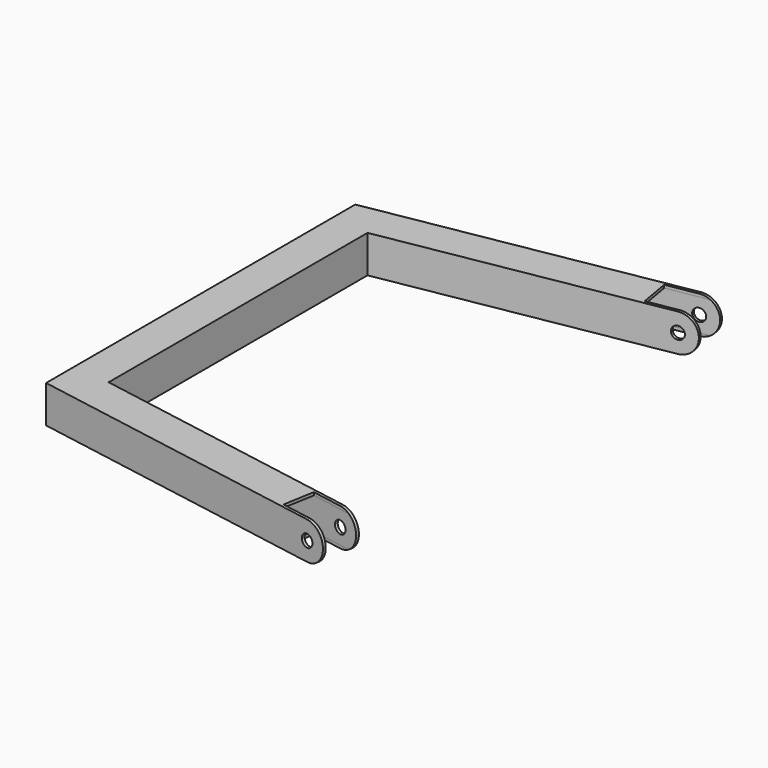
from build123d import *

# Parameters (mm, degrees)
F1_DEPTH  = 19.05
F2_T      = -1.4732
F3_W      = 16.1036
F3_H      = 19.05
F4_DEPTH  = 25.4
F5_R      = 9.52499
F6_R      = 3.175
F7_DEPTH  = 250.7881261572
F8_W      = 16.1036
F8_H      = 19.05
F9_DEPTH  = 25.4
F10_R     = 9.52499
F11_R     = 3.175
F12_DEPTH = 250.7881261572


# Not quite as in the source:
# - a fillet or chamfer is up to 0.001 mm smaller than in the source, because OpenCascade refuses the exact size


with BuildPart() as f1:
    # F0 (on Top) → F1 (new body)
    with BuildSketch(Plane.XY):
        Polygon((0, 225.425), (0, 28.575), (163.8898551464, 0), (167.1619531291, 18.766882394), (19.05, 44.5909277987), (19.05, 209.4090722013), (167.1619531291, 235.233117606), (163.8898551464, 254), align=None)
    extrude(amount=F1_DEPTH)

    # F2
    f2_openings = [f1.faces().sort_by_distance(p)[0] for p in [
        (165.525904, 9.383441, 9.525),
        (165.525904, 244.616559, 9.525),
    ]]
    offset(amount=F2_T, openings=f2_openings, kind=Kind.INTERSECTION)

    # F3 (on face) → F4 (cut)
    with BuildSketch(Plane(origin=(159.0546521525, -27.731958645, 0), x_dir=(0.1717636736, 0.9851381834, 0), z_dir=(0.9851381834, -0.1717636736, 0))):
        with Locations((37.6753235911, 9.525)):
            Rectangle(F3_W, F3_H)
    extrude(amount=-F4_DEPTH, mode=Mode.SUBTRACT)

    # F5 (radius 9.525 in the source; OpenCascade refuses exactly that, so slightly less here)
    f5_edges = [f1.edges().sort_by_distance(p)[0] for p in [
        (164.016376, 0.725653, 19.05),
        (167.035432, 18.04123, 19.05),
        (164.016376, 0.725653, 0),
        (167.035432, 18.04123, 0),
    ]]
    fillet(f5_edges, radius=F5_R)

    # F6 (on face) → F7 (cut, through all)
    with BuildSketch(Plane(origin=(4.8352029939, 27.731958645, 0), x_dir=(0.9851381834, -0.1717636736, 0), z_dir=(-0.1717636736, -0.9851381834, 0))):
        with Locations((151.9291541789, 9.525)):
            Circle(F6_R)
    extrude(amount=-F7_DEPTH, mode=Mode.SUBTRACT)

    # F8 (on face) → F9 (cut)
    with BuildSketch(Plane(origin=(202.0342343209, 35.2256595783, 0), x_dir=(-0.1717636736, 0.9851381834, 0), z_dir=(0.9851381834, 0.1717636736, 0))):
        with Locations((212.5497749961, 9.525)):
            Rectangle(F8_W, F8_H)
    extrude(amount=-F9_DEPTH, mode=Mode.SUBTRACT)

    # F10 (radius 9.525 in the source; OpenCascade refuses exactly that, so slightly less here)
    f10_edges = [f1.edges().sort_by_distance(p)[0] for p in [
        (164.016376, 253.274347, 0),
        (164.016376, 253.274347, 19.05),
        (167.035432, 235.95877, 19.05),
        (167.035432, 235.95877, 0),
    ]]
    fillet(f10_edges, radius=F10_R)

    # F11 (on face) → F12 (cut, through all)
    with BuildSketch(Plane(origin=(-38.1443791745, 218.7743404217, 0), x_dir=(-0.9851381834, -0.1717636736, 0), z_dir=(-0.1717636736, 0.9851381834, 0))):
        with Locations((-195.5571272816, 9.525)):
            Circle(F11_R)
    extrude(amount=-F12_DEPTH, mode=Mode.SUBTRACT)


solid = f1.part
